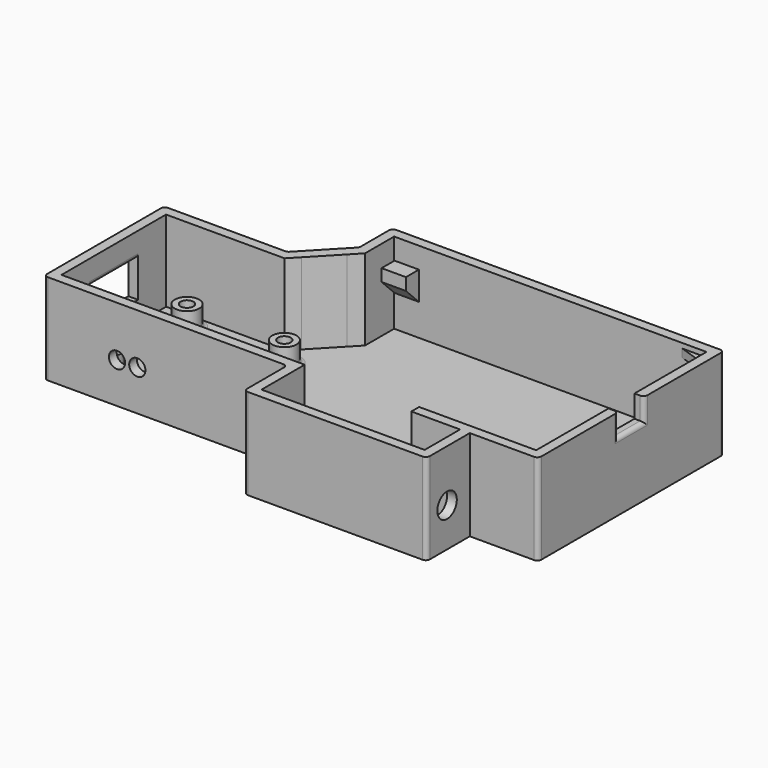
from build123d import *

# Parameters (mm, degrees)
F1_DEPTH       = 25.4
F0_R           = 3.81
F0_W           = 7.62
F0_H           = 5.08
F0_R_2         = 2.0193
F2_DEPTH       = 3.048
F3_DEPTH       = 6.35
F4_R           = 3.81
F5_DEPTH       = 6.35
F6_W           = 4.4349184911
F6_H           = 14.5074356901
F7_DEPTH       = 3.81
F8_W           = 19.05
F8_H           = 11.43
F9_DEPTH       = 5.08
F10_W          = 10.16
F10_H          = 7.112
F11_DEPTH      = 3.175
F13_W          = 7.62
F13_H          = 5.08
F14_DEPTH      = 12.7
F15_T4_DEPTH   = 30.482261763
F15_T9_DEPTH   = 30.482261763
F15_T14_DEPTH  = 30.482261763
F15_2_T1_DEPTH = 53.344523526
F18_DEPTH      = 2.54
F19_R          = 2.54
F20_DEPTH      = 3.048
F21_R          = 1.27


# Not quite as in the source:
# - a fillet or chamfer that OpenCascade refuses, or shapes differently, is made with other operations: its cross-section is extruded or revolved along the edge and cut away or added


with BuildPart() as f1:
    # F0 (on Top) → F1 (new body)
    with BuildSketch(Plane.XY):
        Polygon((30.5370476484, -36.425), (51.925, -36.425), (51.925, 36.2979981456), (-51.925, 36.2979981456), (-51.925, 23.4314990728), (-64.2100349069, 10.565), (-102.725, 10.565), (-102.725, -36.425), (-51.925, -36.425), (-26.6129523516, -36.425), (-26.6129523516, -53.316), (30.5370476484, -53.316), align=None)
        Polygon((-62.5797808525, 7.5170018544), (-59.6695281565, 10.565), (-51.925, 18.6760851618), (-48.8770018544, 21.8683484), (-48.8770018544, 33.25), (-48.75, 33.25), (-41.13, 33.25), (41.2570018544, 33.25), (48.8770018544, 33.25), (48.8770018544, 28.17), (48.8770018544, -28.2970018544), (48.8770018544, -33.3770018544), (41.2570018544, -33.3770018544), (27.4890495028, -33.3770018544), (12.2490495028, -33.3770018544), (12.2490495028, -36.425), (27.4890495028, -36.425), (27.4890495028, -50.2680018544), (-23.564954206, -50.2680018544), (-23.564954206, -33.3770018544), (-51.925, -33.3770018544), (-99.6770018544, -33.3770018544), (-99.6770018544, 7.5170018544), align=None, mode=Mode.SUBTRACT)
    extrude(amount=F1_DEPTH)

    # F0 (on Top) → F2 (join)
    with BuildSketch(Plane.XY):
        Polygon((30.5370476484, -36.425), (51.925, -36.425), (51.925, 36.2979981456), (-51.925, 36.2979981456), (-51.925, 23.4314990728), (-64.2100349069, 10.565), (-102.725, 10.565), (-102.725, -36.425), (-51.925, -36.425), (-26.6129523516, -36.425), (-26.6129523516, -53.316), (30.5370476484, -53.316), align=None)
        Polygon((-62.5797808525, 7.5170018544), (-59.6695281565, 10.565), (-51.925, 18.6760851618), (-48.8770018544, 21.8683484), (-48.8770018544, 33.25), (-48.75, 33.25), (-41.13, 33.25), (41.2570018544, 33.25), (48.8770018544, 33.25), (48.8770018544, 28.17), (48.8770018544, -28.2970018544), (48.8770018544, -33.3770018544), (41.2570018544, -33.3770018544), (27.4890495028, -33.3770018544), (12.2490495028, -33.3770018544), (12.2490495028, -36.425), (27.4890495028, -36.425), (27.4890495028, -50.2680018544), (-23.564954206, -50.2680018544), (-23.564954206, -33.3770018544), (-51.925, -33.3770018544), (-99.6770018544, -33.3770018544), (-99.6770018544, 7.5170018544), align=None, mode=Mode.SUBTRACT)
        Polygon((-51.925, 18.6760851618), (-59.6695281565, 10.565), (-62.5797808525, 7.5170018544), (-99.6770018544, 7.5170018544), (-99.6770018544, -33.3770018544), (-51.925, -33.3770018544), (-23.564954206, -33.3770018544), (-23.564954206, -50.2680018544), (27.4890495028, -50.2680018544), (27.4890495028, -36.425), (12.2490495028, -36.425), (12.2490495028, -33.3770018544), (27.4890495028, -33.3770018544), (41.2570018544, -33.3770018544), (41.2570018544, -28.2970018544), (48.8770018544, -28.2970018544), (48.8770018544, 28.17), (41.2570018544, 28.17), (41.2570018544, 33.25), (-41.13, 33.25), (-41.13, 28.17), (-48.75, 28.17), (-48.75, 33.25), (-48.8770018544, 33.25), (-48.8770018544, 21.8683484), align=None)
        with Locations((-88.9438392901, -28.1826965511)):
            Circle(F0_R, mode=Mode.SUBTRACT)
        with Locations((-58.4638392901, -28.1826965511)):
            Circle(F0_R, mode=Mode.SUBTRACT)
        with Locations((-44.94, -30.71)):
            Rectangle(F0_W, F0_H, mode=Mode.SUBTRACT)
        with Locations((-88.9438392901, 2.2973034489)):
            Circle(F0_R, mode=Mode.SUBTRACT)
        with Locations((-58.4638392901, 2.2973034489)):
            Circle(F0_R, mode=Mode.SUBTRACT)
        with Locations((-58.4638392901, 2.2973034489)):
            Circle(F0_R)
        with Locations((-58.4638392901, 2.2973034489)):
            Circle(F0_R_2, mode=Mode.SUBTRACT)
        with Locations((-88.9438392901, 2.2973034489)):
            Circle(F0_R)
        with Locations((-88.9438392901, 2.2973034489)):
            Circle(F0_R_2, mode=Mode.SUBTRACT)
        with Locations((-58.4638392901, -28.1826965511)):
            Circle(F0_R)
        with Locations((-58.4638392901, -28.1826965511)):
            Circle(F0_R_2, mode=Mode.SUBTRACT)
        with Locations((-88.9438392901, -28.1826965511)):
            Circle(F0_R)
        with Locations((-88.9438392901, -28.1826965511)):
            Circle(F0_R_2, mode=Mode.SUBTRACT)
        with Locations((-44.94, -30.71)):
            Rectangle(F0_W, F0_H)
        with Locations((45.0670018544, -30.8370018544)):
            Rectangle(F0_W, F0_H)
        with Locations((45.0670018544, 30.71)):
            Rectangle(F0_W, F0_H)
        with Locations((-44.94, 30.71)):
            Rectangle(F0_W, F0_H)
        with Locations((-88.9438392901, -28.1826965511)):
            Circle(F0_R_2)
        with Locations((-88.9438392901, 2.2973034489)):
            Circle(F0_R_2)
        with Locations((-58.4638392901, 2.2973034489)):
            Circle(F0_R_2)
        with Locations((-58.4638392901, -28.1826965511)):
            Circle(F0_R_2)
    extrude(amount=-F2_DEPTH)

    # F0 (on Top) → F3 (join)
    with BuildSketch(Plane.XY):
        with Locations((-58.4638392901, 2.2973034489)):
            Circle(F0_R)
        with Locations((-58.4638392901, 2.2973034489)):
            Circle(F0_R_2, mode=Mode.SUBTRACT)
        with Locations((-88.9438392901, 2.2973034489)):
            Circle(F0_R)
        with Locations((-88.9438392901, 2.2973034489)):
            Circle(F0_R_2, mode=Mode.SUBTRACT)
        with Locations((-88.9438392901, -28.1826965511)):
            Circle(F0_R)
        with Locations((-88.9438392901, -28.1826965511)):
            Circle(F0_R_2, mode=Mode.SUBTRACT)
        with Locations((-58.4638392901, -28.1826965511)):
            Circle(F0_R)
        with Locations((-58.4638392901, -28.1826965511)):
            Circle(F0_R_2, mode=Mode.SUBTRACT)
    extrude(amount=F3_DEPTH)

    # F4 (on face) → F5 (cut)
    with BuildSketch(Plane.YZ.offset(30.5370476484)):
        with Locations((-45.315, 9.144)):
            Circle(F4_R)
    extrude(amount=-F5_DEPTH, mode=Mode.SUBTRACT)

    # F6 (on face) → F7 (join)
    with BuildSketch(Plane.XY):
        with Locations((-16.6384097427, -41.2515513599)):
            Rectangle(F6_W, F6_H)
    extrude(amount=F7_DEPTH)

    # F8 (on face) → F9 (cut)
    with BuildSketch(Plane(origin=(-102.725, 0, 0), x_dir=(0, -1, 0), z_dir=(-1, 0, 0))):
        with Locations((12.93, 12.065)):
            Rectangle(F8_W, F8_H)
    extrude(amount=-F9_DEPTH, mode=Mode.SUBTRACT)

    # F10 (on face) → F11 (cut)
    with BuildSketch(Plane.YZ.offset(51.925)):
        with Locations((0, 21.9964)):
            Rectangle(F10_W, F10_H)
    extrude(amount=-F11_DEPTH, mode=Mode.SUBTRACT)

    # F13 (on offset) → F14, piece 2 (join)
    with BuildSketch(Plane.XY.offset(18.796)):
        with Locations((45.0670018544, -30.8370018544)):
            Rectangle(F13_W, F13_H)
        with Locations((-44.94, 30.71)):
            Rectangle(F13_W, F13_H)
        with Locations((45.0670018544, 30.71)):
            Rectangle(F13_W, F13_H)
    extrude(amount=-F14_DEPTH)

    # F15: chamfer of 8.89 on 3 edges, made by hand


with BuildPart() as f14:
    # F13 (on offset) → F14 (new body)
    with BuildSketch(Plane.XY.offset(18.796)):
        with Locations((-44.94, -30.71)):
            Rectangle(F13_W, F13_H)
    extrude(amount=-F14_DEPTH)

    # F15#2: chamfer of 8.89 on 1 edges, made by hand

    # F15_2_s2 → F15_2_t1 (cut)
    with BuildSketch(Plane.YZ.offset(-71.612261763)):
        Polygon((-28.17, 14.986), (-37.06, 6.096), (-28.17, 6.096), align=None)
    extrude(amount=F15_2_T1_DEPTH, mode=Mode.SUBTRACT)


with BuildPart() as f15_tool2:
    # F15_s3 → F15_t4 (new body)
    with BuildSketch(Plane.YZ.offset(-48.75)):
        Polygon((37.06, 6.096), (28.17, 14.986), (28.17, 6.096), align=None)
    extrude(amount=F15_T4_DEPTH)

    split(bisect_by=Plane.XZ.offset(-33.25), keep=Keep.TOP)


with BuildPart() as f1_1:
    add(f1.part)

    # F15_t1: cut F15_tool2
    add(f15_tool2.part, mode=Mode.SUBTRACT)


with BuildPart() as f15_tool7:
    # F15_s8 → F15_t9 (new body)
    with BuildSketch(Plane.YZ.offset(18.3947400914)):
        Polygon((28.17, 14.986), (37.06, 6.096), (28.17, 6.096), align=None)
    extrude(amount=F15_T9_DEPTH)

    split(bisect_by=Plane.XZ.offset(-33.25), keep=Keep.TOP)


with BuildPart() as f1_2:
    add(f1_1.part)

    # F15_t6: cut F15_tool7
    add(f15_tool7.part, mode=Mode.SUBTRACT)


with BuildPart() as f15_tool12:
    # F15_s13 → F15_t14 (new body)
    with BuildSketch(Plane.YZ.offset(48.8770018544)):
        Polygon((-37.1870018544, 6.096), (-28.2970018544, 14.986), (-28.2970018544, 6.096), align=None)
    extrude(amount=-F15_T14_DEPTH)

    split(bisect_by=Plane.XZ.offset(33.3770018544), keep=Keep.BOTTOM)


with BuildPart() as f1_3:
    add(f1_2.part)

    # F15_t11: cut F15_tool12
    add(f15_tool12.part, mode=Mode.SUBTRACT)

    # F17 (on offset) → F18 (join)
    with BuildSketch(Plane.XY.offset(21.336)):
        Polygon((41.2570018544, -33.3770018544), (48.8770018544, -33.3770018544), (48.8770018544, -30.8370018544), align=None)
        Polygon((41.2570018544, 33.25), (48.8770018544, 30.71), (48.8770018544, 33.25), align=None)
    extrude(amount=F18_DEPTH)

    # F19 (on face) → F20 (cut)
    with BuildSketch(Plane.XZ.offset(36.425)):
        with Locations((-79.865, 9.652)):
            Circle(F19_R)
        with Locations((-73.515, 9.652)):
            Circle(F19_R)
    extrude(amount=-F20_DEPTH, mode=Mode.SUBTRACT)

    # F21
    f21_edges = [f1_3.edges().sort_by_distance(p)[0] for p in [
        (51.925, -36.425, 11.176),
        (30.537048, -53.316, 11.176),
        (-26.612952, -53.316, 11.176),
        (-26.612952, -36.425, 11.176),
        (-102.725, -36.425, 11.176),
        (-102.725, 10.565, 11.176),
        (-64.210035, 10.565, 11.176),
        (-51.925, 23.431499, 11.176),
        (-51.925, 36.297998, 11.176),
        (51.925, 36.297998, 11.176),
        (-62.273839, -28.182697, 0),
        (-92.753839, -28.182697, 0),
        (-62.273839, 2.297303, 0),
        (-92.753839, 2.297303, 0),
        (51.925, -5.08, 21.9202),
        (51.925, 0, 18.4404),
        (51.925, 5.08, 21.9202),
        (-99.677002, -12.93, 17.78),
    ]]
    fillet(f21_edges, radius=F21_R)


solid = Compound([f14.part, f1_3.part])
